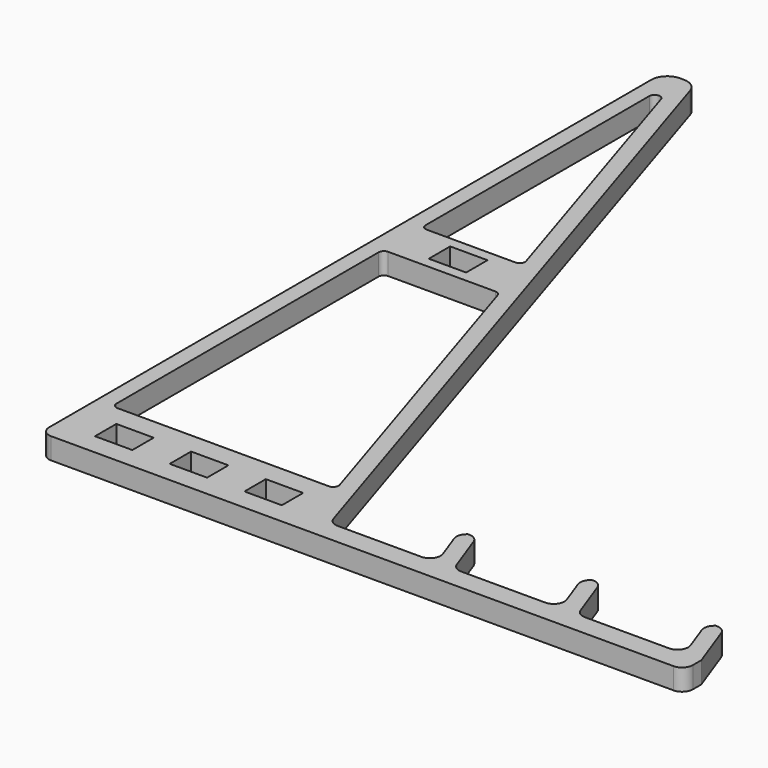
from build123d import *

# Parameters (mm, degrees)
F0_W        = 7
F0_H        = 5
F1_DEPTH    = 4
F2_T1_DEPTH = 4
F2_T3_DEPTH = 14


# Not quite as in the source:
# - a fillet or chamfer that OpenCascade refuses, or shapes differently, is made with other operations: its cross-section is extruded or revolved along the edge and cut away or added
# - a feature names something its author has since deleted; it is built from what else it names


with BuildPart() as f1:
    # F0 (on Top) → F1 (new body)
    with BuildSketch(Plane.XY):
        with BuildLine():
            Line((-51, 139), (-51, -4))
            Line((-51, -4), (69.5775999523, -4))
            Line((69.5775999523, -4), (69.5775999523, 0))
            Line((69.5775999523, 0), (66.3850666349, 0))
            Line((66.3850666349, 0), (46.3850666349, 0))
            Line((46.3850666349, 0), (43.1925333174, 0))
            Line((43.1925333174, 0), (23.1925333174, 0))
            Line((23.1925333174, 0), (20, 0))
            Line((20, 0), (0, 0))
            Line((0, 0), (-44.4302483166, 139.9080159757))
            ThreePointArc((-44.4302483166, 139.9080159757), (-45.5180993372, 141.4211616971), (-47.2895326655, 142))
            Line((-47.2895326655, 142), (-48, 142))
            ThreePointArc((-48, 142), (-50.1213203436, 141.1213203436), (-51, 139))
        make_face()
        with Locations((-40.5, 2.5)):
            Rectangle(F0_W, F0_H, mode=Mode.SUBTRACT)
        with Locations((-26.5, 2.5)):
            Rectangle(F0_W, F0_H, mode=Mode.SUBTRACT)
        with Locations((-12.5, 2.5)):
            Rectangle(F0_W, F0_H, mode=Mode.SUBTRACT)
        with BuildLine():
            Line((-7.3725300405, 9), (-47, 9))
            ThreePointArc((-47, 9), (-47.7071067812, 9.2928932188), (-48, 10))
            Line((-48, 10), (-48, 71.4074290533))
            ThreePointArc((-48, 71.4074290533), (-47.7071067812, 72.1145358345), (-47, 72.4074290533))
            Line((-47, 72.4074290533), (-26.8735379155, 72.4074290533))
            ThreePointArc((-26.8735379155, 72.4074290533), (-26.2830601394, 72.2144829523), (-25.9204431326, 71.7101010452))
            Line((-25.9204431326, 71.7101010452), (-6.4194352575, 10.3026719919))
            ThreePointArc((-6.4194352575, 10.3026719919), (-6.5654761415, 9.4095222239), (-7.3725300405, 9))
        make_face(mode=Mode.SUBTRACT)
        with Locations((-37.5, 76.9074290533)):
            Rectangle(F0_W, F0_H, mode=Mode.SUBTRACT)
        with BuildLine():
            ThreePointArc((-48, 134.7843734895), (-47.1531424452, 135.7725776139), (-46.046905217, 135.0870454814))
            Line((-46.046905217, 135.0870454814), (-29.4136863758, 82.7101010452))
            ThreePointArc((-29.4136863758, 82.7101010452), (-29.5597272597, 81.8169512772), (-30.3667811588, 81.4074290533))
            Line((-30.3667811588, 81.4074290533), (-47, 81.4074290533))
            ThreePointArc((-47, 81.4074290533), (-47.7071067812, 81.7003222721), (-48, 82.4074290533))
            Line((-48, 82.4074290533), (-48, 134.7843734895))
        make_face(mode=Mode.SUBTRACT)
        Polygon((66.3850666349, 0), (69.5775999523, 0), (65.783943064, 10.4229866378), (62.9648652016, 9.3969262079), align=None)
        Polygon((43.1925333174, 0), (46.3850666349, 0), (42.5914097465, 10.4229866378), (39.7723318842, 9.3969262079), align=None)
        Polygon((16.5797985667, 9.3969262079), (20, 0), (23.1925333174, 0), (19.3988764291, 10.4229866378), align=None)
    extrude(amount=F1_DEPTH)

    # F2: fillet of radius 2 on 14 edges, made by hand

    # F2_s2 → F2_t1 (join)
    with BuildSketch(Plane.XY):
        with BuildLine():
            ThreePointArc((42.2156225455, 2.6840402867), (41.9745413925, 0.8528471273), (40.3362373039, 0))
            Line((40.3362373039, 0), (43.1925333174, 0))
            Line((43.1925333174, 0), (42.2156225455, 2.6840402867))
        make_face()
        with BuildLine():
            ThreePointArc((47.7854817113, 0), (46.6383288386, 0.3616959114), (45.9060964697, 1.3159597133))
            Line((45.9060964697, 1.3159597133), (46.3850666349, 0))
            Line((46.3850666349, 0), (47.7854817113, 0))
        make_face()
        with BuildLine():
            ThreePointArc((65.4081558629, 2.6840402867), (65.1670747099, 0.8528471273), (63.5287706214, 0))
            Line((63.5287706214, 0), (66.3850666349, 0))
            Line((66.3850666349, 0), (65.4081558629, 2.6840402867))
        make_face()
        with BuildLine():
            ThreePointArc((24.5929483938, 0), (23.4457955211, 0.3616959114), (22.7135631523, 1.3159597133))
            Line((22.7135631523, 1.3159597133), (23.1925333174, 0))
            Line((23.1925333174, 0), (24.5929483938, 0))
        make_face()
        with BuildLine():
            ThreePointArc((19.0230892281, 2.6840402867), (18.7820080751, 0.8528471273), (17.1437039865, 0))
            Line((17.1437039865, 0), (20, 0))
            Line((20, 0), (19.0230892281, 2.6840402867))
        make_face()
        with BuildLine():
            ThreePointArc((1.4632920473, 0), (0.2823364951, 0.3858922019), (-0.4428975187, 1.3946560162))
            Line((-0.4428975187, 1.3946560162), (0, 0))
            Line((0, 0), (1.4632920473, 0))
        make_face()
    extrude(amount=F2_T1_DEPTH)

    # F2_s4 → F2_t3 (cut)
    with BuildSketch(Plane.XY.offset(-5)):
        with BuildLine():
            ThreePointArc((66.4679833506, 8.5436013963), (65.4338346325, 9.6721766837), (63.9045578224, 9.7389463512))
            Line((63.9045578224, 9.7389463512), (65.783943064, 10.4229866378))
            Line((65.783943064, 10.4229866378), (66.4679833506, 8.5436013963))
        make_face()
        with BuildLine():
            ThreePointArc((64.8442504432, 10.0809664945), (63.7156751557, 9.0468177764), (63.6489054883, 7.5175409663))
            Line((63.6489054883, 7.5175409663), (62.9648652016, 9.3969262079))
            Line((62.9648652016, 9.3969262079), (64.8442504432, 10.0809664945))
        make_face()
        with BuildLine():
            ThreePointArc((20.0829167158, 8.5436013963), (19.0487679977, 9.6721766837), (17.5194911875, 9.7389463512))
            Line((17.5194911875, 9.7389463512), (19.3988764291, 10.4229866378))
            Line((19.3988764291, 10.4229866378), (20.0829167158, 8.5436013963))
        make_face()
        with BuildLine():
            ThreePointArc((18.4591838083, 10.0809664945), (17.3306085209, 9.0468177764), (17.2638388534, 7.5175409663))
            Line((17.2638388534, 7.5175409663), (16.5797985667, 9.3969262079))
            Line((16.5797985667, 9.3969262079), (18.4591838083, 10.0809664945))
        make_face()
        with BuildLine():
            ThreePointArc((41.6517171257, 10.0809664945), (40.5231418383, 9.0468177764), (40.4563721708, 7.5175409663))
            Line((40.4563721708, 7.5175409663), (39.7723318842, 9.3969262079))
            Line((39.7723318842, 9.3969262079), (41.6517171257, 10.0809664945))
        make_face()
        with BuildLine():
            ThreePointArc((43.2754500332, 8.5436013963), (42.2413013151, 9.6721766837), (40.712024505, 9.7389463512))
            Line((40.712024505, 9.7389463512), (42.5914097465, 10.4229866378))
            Line((42.5914097465, 10.4229866378), (43.2754500332, 8.5436013963))
        make_face()
        with BuildLine():
            ThreePointArc((67.5775999523, -4), (68.9918135147, -3.4142135624), (69.5775999523, -2))
            Line((69.5775999523, -2), (69.5775999523, -4))
            Line((69.5775999523, -4), (67.5775999523, -4))
        make_face()
        with BuildLine():
            ThreePointArc((-51, -2), (-50.4142135624, -3.4142135624), (-49, -4))
            Line((-49, -4), (-51, -4))
            Line((-51, -4), (-51, -2))
        make_face()
    extrude(amount=F2_T3_DEPTH, mode=Mode.SUBTRACT)


solid = f1.part
